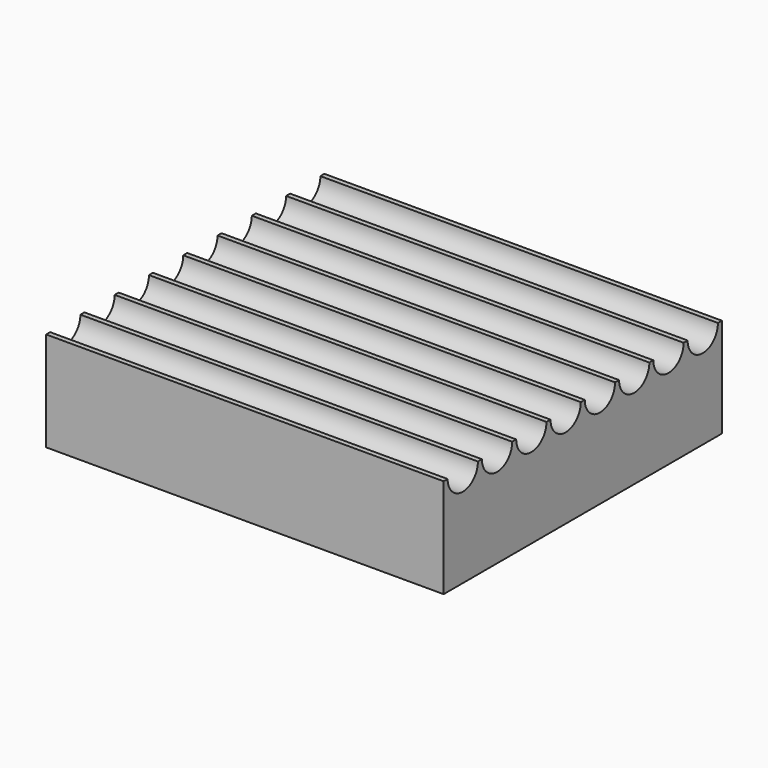
from build123d import *

# Parameters (mm, degrees)
F0_W     = 12.7
F0_H     = 11.1125
F1_DEPTH = 6.35
F2_R     = 0.6047619048
F3_DEPTH = 12.701
F4_DEPTH = 3.175


# Not quite as in the source:
# - a length typed as a fraction of an inch, garbled in the dataset ("3 / 203.2 mm" for 3/8 in), is restored


with BuildPart() as f1:
    # F0 (on Top) → F1 (new body)
    with BuildSketch(Plane.XY):
        with Locations((6.35, 5.55625)):
            Rectangle(F0_W, F0_H)
    extrude(amount=F1_DEPTH)

    # F2 (on face) → F3 (cut, through all)
    with BuildSketch(Plane(origin=(0, 0, 0), x_dir=(0, -1, 0), z_dir=(-1, 0, 0))):
        with Locations((-10.3481481481, 3.175)):
            Circle(F2_R)
        with Locations((-8.9790343915, 3.175)):
            Circle(F2_R)
        with Locations((-7.6099206349, 3.175)):
            Circle(F2_R)
        with Locations((-6.2408068783, 3.175)):
            Circle(F2_R)
        with Locations((-4.8716931217, 3.175)):
            Circle(F2_R)
        with Locations((-3.5025793651, 3.175)):
            Circle(F2_R)
        with Locations((-2.1334656085, 3.175)):
            Circle(F2_R)
        with Locations((-0.7643518519, 3.175)):
            Circle(F2_R)
    extrude(amount=-F3_DEPTH, mode=Mode.SUBTRACT)

    # F4 (cut): a face of the model
    f4_faces = [f1.faces().sort_by_distance(p)[0] for p in [
        (6.35, 5.55625, 6.35),
    ]]
    extrude(f4_faces, amount=-F4_DEPTH, mode=Mode.SUBTRACT)


solid = f1.part
